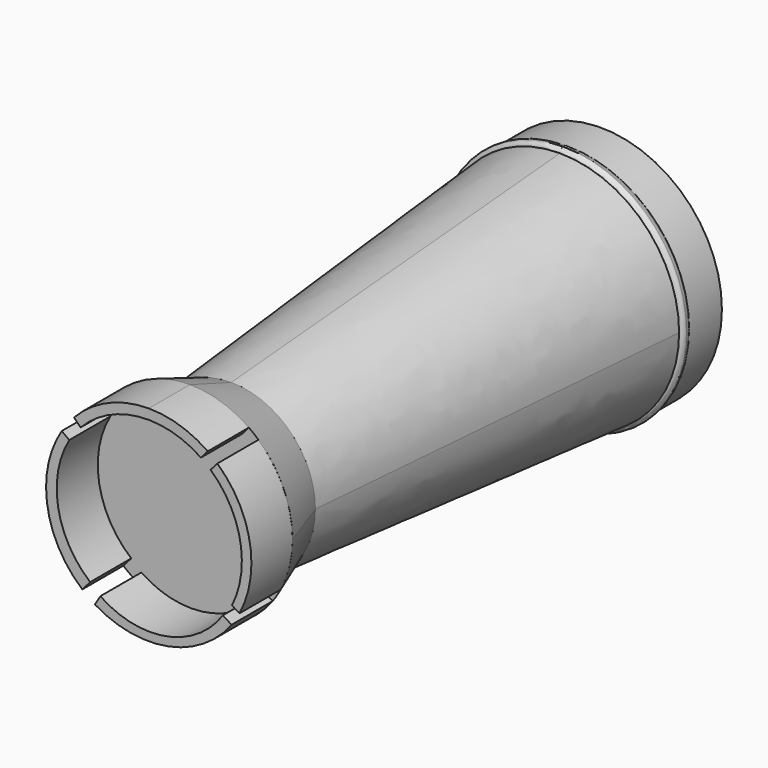
from build123d import *

# Parameters (mm, degrees)
F0_R      = 149.4225994351
F1_DEPTH  = 50.8
F2_R      = 152.4
F2_R_2    = 149.4225994351
F3_DEPTH  = 12.7
F5_R      = 5.08
F3_FACE_R = 147.32
F10_R     = 127
F13_DEPTH = 63.5


# Not quite as in the source:
# - a fillet or chamfer that OpenCascade refuses, or shapes differently, is made with other operations: its cross-section is extruded or revolved along the edge and cut away or added
# - ends of sketch curves that miss each other by under 0.0002 mm in the source are joined


with BuildPart() as f1:
    # F0 (on Front) → F1 (new body)
    with BuildSketch(Plane.XZ):
        with Locations((-292.8719222546, -169.214874506)):
            Circle(F0_R)
    extrude(amount=F1_DEPTH)

    # F2 (on face) → F3 (join)
    with BuildSketch(Plane.XZ.offset(50.8)):
        with Locations((-292.8719222546, -169.214874506)):
            Circle(F2_R)
        with Locations((-292.8719222546, -169.214874506)):
            Circle(F2_R_2, mode=Mode.SUBTRACT)
        with Locations((-292.8719222546, -169.214874506)):
            Circle(F2_R_2)
    extrude(amount=F3_DEPTH)

    # F4: fillet of radius 10.16 on 1 edges, made by hand

    # F4_s1 → F4_t2 (revolve, cut)
    with BuildSketch(Plane.XY.offset(-169.214874506)):
        with BuildLine():
            ThreePointArc((-140.4715222546, -57.9862101152), (-141.2453680799, -54.0967598366), (-143.4490400288, -50.7997171052))
            Line((-143.4490400288, -50.7997171052), (-142.7306552377, -50.0810678042))
            ThreePointArc((-142.7306552377, -50.0810678042), (-141.9604811417, -49.7838634315), (-140.4719222546, -49.7838634315))
            Line((-140.4719222546, -49.7838634315), (-139.455785686, -50.8))
            ThreePointArc((-139.455785686, -50.8), (-139.455785686, -54.3931050576), (-139.455385686, -57.9862101152))
            Line((-139.455385686, -57.9862101152), (-140.4715222546, -57.9862101152))
        make_face()
    revolve(axis=Axis((-292.8719222546, -50.8, -169.214874506), (0, -1, 0)), mode=Mode.SUBTRACT)

    # F5
    f5_edges = [f1.edges().sort_by_distance(p)[0] for p in [
        (-445.271922, -63.5, -169.214875),
    ]]
    fillet(f5_edges, radius=F5_R)


with BuildPart() as f8:
    # F3_face (on face) → F8 section 0
    with BuildSketch(Plane(origin=(-292.8719222546, -63.5, -169.214874506), x_dir=(1, 0, 0), z_dir=(0, -1, 0))):
        Circle(F3_FACE_R)
    # F7 (on offset) → F8 section 1
    with BuildSketch(Plane.XZ.offset(571.5)):
        with BuildLine():
            ThreePointArc((-188.8432323815, -168.8047898933), (-219.3094074441, -95.2529368637), (-292.8612604737, -64.7867618011))
            ThreePointArc((-292.8612604737, -64.7867618011), (-366.4131135034, -95.2529368637), (-396.8792885659, -168.8047898933))
            ThreePointArc((-396.8792885659, -168.8047898933), (-366.4131135034, -242.356642923), (-292.8612604737, -272.8228179855))
            ThreePointArc((-292.8612604737, -272.8228179855), (-219.3094074441, -242.356642923), (-188.8432323815, -168.8047898933))
        make_face()
    loft()

    # F8_face (on face) → F11 section 0
    with BuildSketch(Plane(origin=(-292.8612604737, -571.5, -168.8047898933), x_dir=(1, 0, 0), z_dir=(0, -1, 0))):
        with BuildLine():
            ThreePointArc((104.0180280922, 0), (73.5518530297, 73.5518530297), (0, 104.0180280922))
            ThreePointArc((0, 104.0180280922), (-73.5518530297, 73.5518530297), (-104.0180280922, 0))
            ThreePointArc((-104.0180280922, 0), (-73.5518530297, -73.5518530297), (0, -104.0180280922))
            ThreePointArc((0, -104.0180280922), (73.5518530297, -73.5518530297), (104.0180280922, 0))
        make_face()
    # F10 (on offset) → F11 section 1
    with BuildSketch(Plane.XZ.offset(635)):
        with Locations((-293.2986815244, -168.6145133888)):
            Circle(F10_R)
    loft()

    # F12 (on face) → F13 (join)
    with BuildSketch(Plane.XZ.offset(635)):
        with BuildLine():
            Line((-391.5979862213, -108.0022379756), (-400.9201721133, -101.1858012074))
            ThreePointArc((-400.9201721133, -101.1858012074), (-415.3579569892, -133.5354651206), (-420.2986816338, -168.6145133888))
            ThreePointArc((-420.2986816338, -168.6145133888), (-408.5621527866, -221.9374064899), (-375.5218381286, -265.4048039891))
            Line((-375.5218381286, -265.4048039891), (-365.7894134521, -254.2508244514))
            ThreePointArc((-365.7894134521, -254.2508244514), (-405.4049768836, -185.8402857464), (-391.5979862213, -108.0022379756))
        make_face()
        with BuildLine():
            Line((-228.8054376841, -74.2525681853), (-220.400493443, -64.6199659103))
            ThreePointArc((-220.400493443, -64.6199659103), (-255.0776205161, -47.5023507464), (-293.2986815244, -41.6145133381))
            ThreePointArc((-293.2986815244, -41.6145133381), (-343.6895158778, -52.0393579803), (-385.8076700214, -81.6024204768))
            Line((-385.8076700214, -81.6024204768), (-377.5976598218, -89.7625237741))
            ThreePointArc((-377.5976598218, -89.7625237741), (-306.0480228678, -54.7003621275), (-228.8054376841, -74.2525681853))
        make_face()
        with BuildLine():
            ThreePointArc((-360.0188401366, -276.6767202506), (-269.1895671051, -292.8597111858), (-191.0046766799, -243.8804406295))
            Line((-191.0046766799, -243.8804406295), (-201.6733586788, -237.045109272))
            ThreePointArc((-201.6733586788, -237.045109272), (-271.5563278796, -282.6318647221), (-353.216022253, -265.5007243156))
            Line((-353.216022253, -265.5007243156), (-360.0188401366, -276.6767202506))
        make_face()
        with BuildLine():
            Line((-216.7594547282, -83.717933659), (-208.5417613742, -74.0349839049))
            Line((-208.5417613742, -74.0349839049), (-216.8890916963, -83.6015569533))
            ThreePointArc((-216.8890916963, -83.6015569533), (-216.8242512933, -83.6597208898), (-216.7594547282, -83.717933659))
        make_face()
        with BuildLine():
            ThreePointArc((-181.2027964678, -228.3096766694), (-168.3558734214, -146.4733672465), (-208.5417613742, -74.0349839049))
            Line((-208.5417613742, -74.0349839049), (-216.7594547282, -83.717933659))
            ThreePointArc((-216.7594547282, -83.717933659), (-180.2895464174, -148.679856079), (-190.4234737158, -222.4864214659))
            Line((-190.4234737158, -222.4864214659), (-181.2027964678, -228.3096766694))
        make_face()
    extrude(amount=F13_DEPTH)


solid = Compound([f1.part, f8.part])
